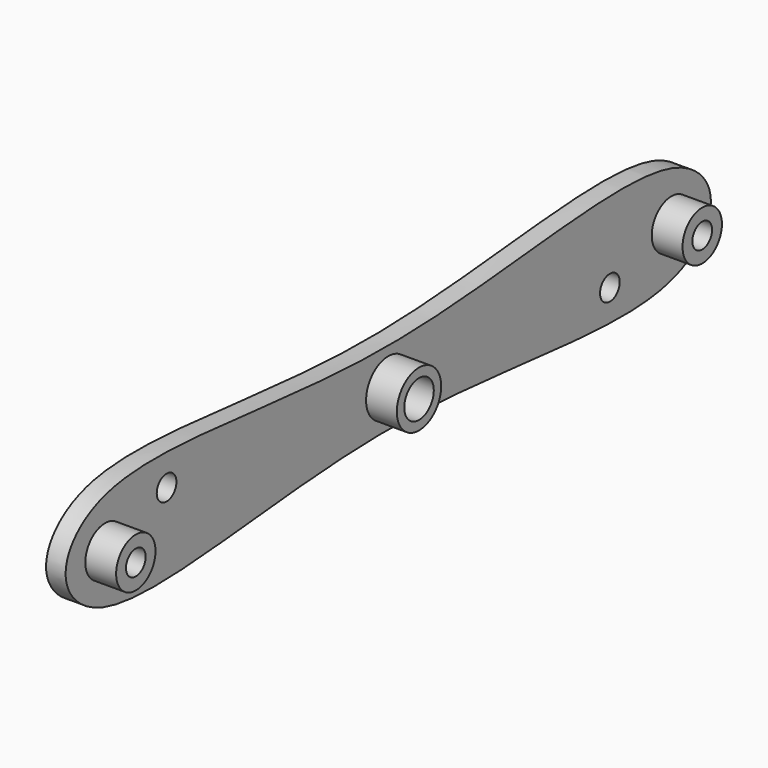
from build123d import *
from build123d import SkipClean  # not in build123d's __all__

# Parameters (mm, degrees)
F0_R     = 4
F1_DEPTH = 6.35
F2_R     = 9
F2_R_2   = 6
F2_R_3   = 8
F2_R_4   = 4
F3_DEPTH = 10
F4_DEPTH = 17
F5_R     = 6
F5_R_2   = 4.25
F6_DEPTH = 5
F7_R     = 4
F8_DEPTH = 25


# Not quite as in the source:
# - after a boolean that leaves OpenCascade's solid faulty, fix() repairs it


with BuildPart() as f1:
    # F0 (on Right) → F1 (new body)
    with BuildSketch(Plane.YZ):
        with BuildLine():
            add(Edge.make_bspline(
                [(-131, 0), (-131, 6.4889437082), (-112.2697628073, 27.6109999607), (0, 1.1848825406), (112.2697628073, 27.6109999607), (136.7541488069, 0), (112.2697628073, -27.6109999607), (0, -1.1848825406), (-112.2697628073, -27.6109999607), (-131, -6.4889437082), (-131, 0)],
                knots=[0, 0, 0, 0, 0.0768029356, 0.25, 0.4231970644, 0.5, 0.5768029356, 0.75, 0.9231970644, 1, 1, 1, 1], degree=3))
        make_face()
        with Locations((-115, 0)):
            Circle(F0_R, mode=Mode.SUBTRACT)
        with BuildLine():
            ThreePointArc((6, 0), (0, -6), (-6, 0))
            ThreePointArc((-6, 0), (0, 6), (6, 0))
        make_face(mode=Mode.SUBTRACT)
        with BuildLine():
            ThreePointArc((119, 0), (115, -4), (111, 0))
            ThreePointArc((111, 0), (115, 4), (119, 0))
        make_face(mode=Mode.SUBTRACT)
    extrude(amount=F1_DEPTH)

    # F2 (on face) → F3 (join)
    with BuildSketch(Plane.YZ.offset(6.35)):
        Circle(F2_R)
        Circle(F2_R_2, mode=Mode.SUBTRACT)
        with Locations((-115, 0)):
            Circle(F2_R_3)
        with Locations((-115, 0)):
            Circle(F2_R_4, mode=Mode.SUBTRACT)
        with Locations((115, 0)):
            Circle(F2_R_3)
        with Locations((115, 0)):
            Circle(F2_R_4, mode=Mode.SUBTRACT)
    with SkipClean():  # cleaning this boolean's faces spoils the solid; the shape is the same uncleaned
        extrude(amount=F3_DEPTH)

    # F4 (add): a face of the model
    f4_faces = [f1.faces().sort_by_distance(p)[0] for p in [
        (16.35, -8.7454415588, 0),
    ]]
    extrude(f4_faces, amount=-F4_DEPTH)

    add(f1.part.fix(), mode=Mode.REPLACE)

    # F5 (on face) → F6 (join)
    with BuildSketch(Plane(origin=(-0.65, 0, 0), x_dir=(0, -1, 0), z_dir=(-1, 0, 0))):
        Circle(F5_R)
        Circle(F5_R_2, mode=Mode.SUBTRACT)
    extrude(amount=-F6_DEPTH)

    # F7 (on face) → F8 (cut)
    with BuildSketch(Plane(origin=(0, 0, 0), x_dir=(0, -1, 0), z_dir=(-1, 0, 0))):
        with Locations((90, 8)):
            Circle(F7_R)
        with Locations((-90, -8)):
            Circle(F7_R)
    extrude(amount=-F8_DEPTH, mode=Mode.SUBTRACT)


solid = f1.part
